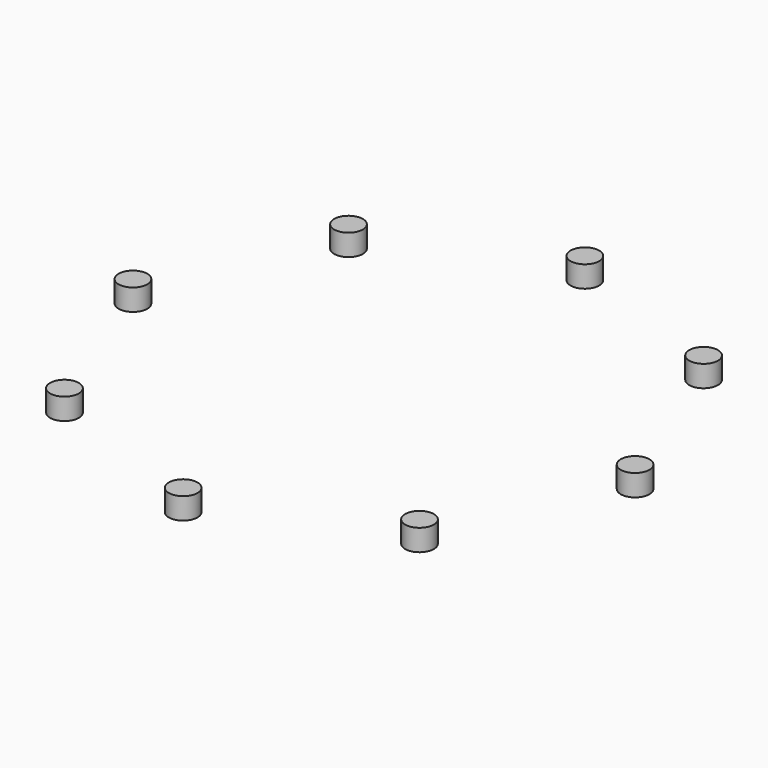
from build123d import *

# Parameters (mm, degrees)
F2_R     = 2
F3_DEPTH = 3


# Not quite as in the source:
# - a feature of the source that left no trace in its solid (it failed there, or was rolled back) is left out
# - the program builds the solid bodies; features that only make, move or delete a surface that nothing else refers to are left out


with BuildPart() as f3:
    # F2 (on face) → F3 (new body)
    with BuildSketch(Plane(origin=(0, 0, -5), x_dir=(1, 0, 0), z_dir=(0, 0, -1))):
        with Locations((0, -35)):
            Circle(F2_R)
    extrude(amount=-F3_DEPTH)


with BuildPart() as f3b:
    # F2 (on face) → F3, piece 2 (new body)
    with BuildSketch(Plane(origin=(0, 0, -5), x_dir=(1, 0, 0), z_dir=(0, 0, -1))):
        with Locations((24.7487373415, -24.7487373415)):
            Circle(F2_R)
    extrude(amount=-F3_DEPTH)


with BuildPart() as f3c:
    # F2 (on face) → F3, piece 3 (new body)
    with BuildSketch(Plane(origin=(0, 0, -5), x_dir=(1, 0, 0), z_dir=(0, 0, -1))):
        with Locations((35, 0)):
            Circle(F2_R)
    extrude(amount=-F3_DEPTH)


with BuildPart() as f3d:
    # F2 (on face) → F3, piece 4 (new body)
    with BuildSketch(Plane(origin=(0, 0, -5), x_dir=(1, 0, 0), z_dir=(0, 0, -1))):
        with Locations((24.7487373415, 24.7487373415)):
            Circle(F2_R)
    extrude(amount=-F3_DEPTH)


with BuildPart() as f3e:
    # F2 (on face) → F3, piece 5 (new body)
    with BuildSketch(Plane(origin=(0, 0, -5), x_dir=(1, 0, 0), z_dir=(0, 0, -1))):
        with Locations((0, 35)):
            Circle(F2_R)
    extrude(amount=-F3_DEPTH)


with BuildPart() as f3f:
    # F2 (on face) → F3, piece 6 (new body)
    with BuildSketch(Plane(origin=(0, 0, -5), x_dir=(1, 0, 0), z_dir=(0, 0, -1))):
        with Locations((-24.7487373415, 24.7487373415)):
            Circle(F2_R)
    extrude(amount=-F3_DEPTH)


with BuildPart() as f3g:
    # F2 (on face) → F3, piece 7 (new body)
    with BuildSketch(Plane(origin=(0, 0, -5), x_dir=(1, 0, 0), z_dir=(0, 0, -1))):
        with Locations((-35, 0)):
            Circle(F2_R)
    extrude(amount=-F3_DEPTH)


with BuildPart() as f3h:
    # F2 (on face) → F3, piece 8 (new body)
    with BuildSketch(Plane(origin=(0, 0, -5), x_dir=(1, 0, 0), z_dir=(0, 0, -1))):
        with Locations((-24.7487373415, -24.7487373415)):
            Circle(F2_R)
    extrude(amount=-F3_DEPTH)


solid = Compound([f3.part, f3b.part, f3c.part, f3d.part, f3e.part, f3f.part, f3g.part, f3h.part])
